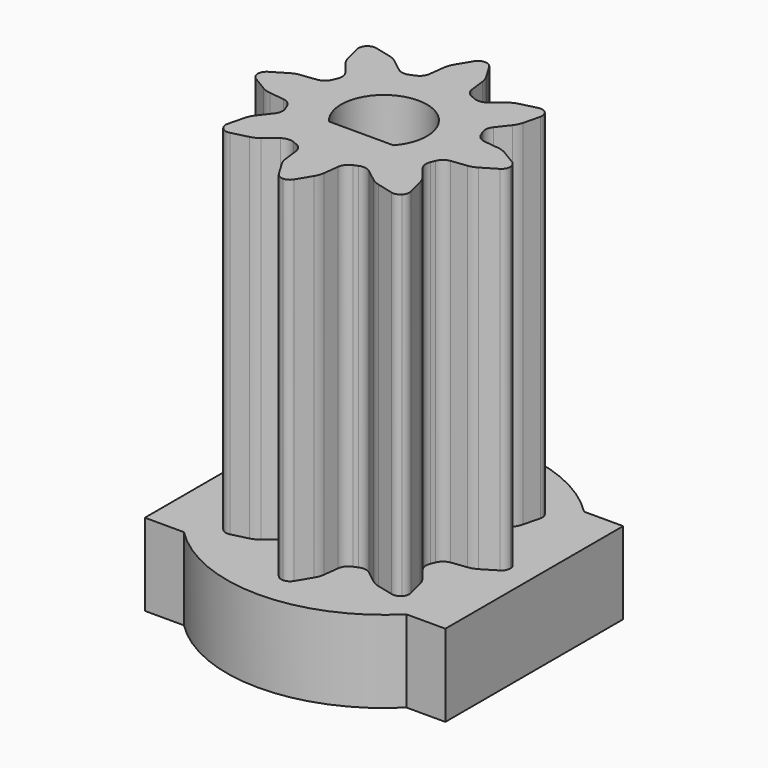
from build123d import *

# Parameters (mm, degrees)
F0_R     = 5
F0_R_2   = 3.15
F0_R_3   = 2.55
F1_DEPTH = 3.25
F2_R     = 2.55
F3_DEPTH = 14


# Not quite as in the source:
# - a feature names something its author has since deleted; it is built from what else it names


with BuildPart() as f1:
    # F0 (on Top) → F1 (new body)
    with BuildSketch(Plane.XY):
        with BuildLine():
            Line((-5.95, -4.4), (-4.4034787385, -4.4))
            ThreePointArc((-4.4034787385, -4.4), (0, -6.225), (4.4034787385, -4.4))
            Line((4.4034787385, -4.4), (5.95, -4.4))
            Line((5.95, -4.4), (5.95, 4.4))
            Line((5.95, 4.4), (4.4034787385, 4.4))
            ThreePointArc((4.4034787385, 4.4), (0, 6.225), (-4.4034787385, 4.4))
            Line((-4.4034787385, 4.4), (-5.95, 4.4))
            Line((-5.95, 4.4), (-5.95, -4.4))
        make_face()
        Circle(F0_R, mode=Mode.SUBTRACT)
        Circle(F0_R)
        Circle(F0_R_2, mode=Mode.SUBTRACT)
        Circle(F0_R_2)
        Circle(F0_R_3, mode=Mode.SUBTRACT)
        Circle(F0_R_3)
        with BuildLine():
            ThreePointArc((-1.275, -1.1244443072), (-0.601040764, 1.5902043894), (1.7, 0))
            ThreePointArc((1.7, 0), (1.5902043894, -0.601040764), (1.275, -1.1244443072))
            ThreePointArc((1.275, -1.1244443072), (0, -1.7), (-1.275, -1.1244443072))
        make_face(mode=Mode.SUBTRACT)
        with BuildLine():
            Line((1.275, -1.1244443072), (-1.275, -1.1244443072))
            ThreePointArc((-1.275, -1.1244443072), (0, -1.7), (1.275, -1.1244443072))
        make_face()
    extrude(amount=F1_DEPTH)

    # F2 (on face) → F3 (join)
    with BuildSketch(Plane.XY.offset(3.25)):
        with BuildLine():
            ThreePointArc((-4.8302633262, 0.3000085552), (-4.9546244936, 0.172348246), (-5, 0))
            ThreePointArc((-5, 0), (-4.9546244936, -0.172348246), (-4.8302633262, -0.3000085552))
            Line((-4.8302633262, -0.3000085552), (-4.2601369618, -0.6425750355))
            ThreePointArc((-4.2601369618, -0.6425750355), (-4.0929165173, -0.7205512094), (-3.9131380826, -0.7620563314))
            Line((-3.9131380826, -0.7620563314), (-3.3117988826, -0.835891501))
            ThreePointArc((-3.3117988826, -0.835891501), (-3.0868883315, -0.9291389359), (-2.9422567869, -1.125))
            ThreePointArc((-2.9422567869, -1.125), (-3.15, 0), (-2.9422567869, 1.125))
            ThreePointArc((-2.9422567869, 1.125), (-3.0868883315, 0.9291389359), (-3.3117988826, 0.835891501))
            Line((-3.3117988826, 0.835891501), (-3.9131380826, 0.7620563314))
            ThreePointArc((-3.9131380826, 0.7620563314), (-4.0929165173, 0.7205512094), (-4.2601369618, 0.6425750355))
            Line((-4.2601369618, 0.6425750355), (-4.8302633262, 0.3000085552))
        make_face()
        with BuildLine():
            ThreePointArc((-3.2033738691, 3.6276500367), (-3.3815799641, 3.6253171911), (-3.5355339059, 3.5355339059))
            ThreePointArc((-3.5355339059, 3.5355339059), (-3.6253171911, 3.3815799641), (-3.6276500367, 3.2033738691))
            Line((-3.6276500367, 3.2033738691), (-3.4667408995, 2.5580025694))
            ThreePointArc((-3.4667408995, 2.5580025694), (-3.4036356706, 2.3846223779), (-3.3058616735, 2.2281512744))
            Line((-3.3058616735, 2.2281512744), (-2.9328599965, 1.7507308991))
            ThreePointArc((-2.9328599965, 1.7507308991), (-2.8397601142, 1.5257592297), (-2.8759848548, 1.2849945972))
            ThreePointArc((-2.8759848548, 1.2849945972), (-2.2273863607, 2.2273863607), (-1.2849945972, 2.8759848548))
            ThreePointArc((-1.2849945972, 2.8759848548), (-1.5257592297, 2.8397601142), (-1.7507308991, 2.9328599965))
            Line((-1.7507308991, 2.9328599965), (-2.2281512744, 3.3058616735))
            ThreePointArc((-2.2281512744, 3.3058616735), (-2.3846223779, 3.4036356706), (-2.5580025694, 3.4667408995))
            Line((-2.5580025694, 3.4667408995), (-3.2033738691, 3.6276500367))
        make_face()
        with BuildLine():
            ThreePointArc((0.3000085552, 4.8302633262), (0.172348246, 4.9546244936), (0, 5))
            ThreePointArc((0, 5), (-0.172348246, 4.9546244936), (-0.3000085552, 4.8302633262))
            Line((-0.3000085552, 4.8302633262), (-0.6425750355, 4.2601369618))
            ThreePointArc((-0.6425750355, 4.2601369618), (-0.7205512094, 4.0929165173), (-0.7620563314, 3.9131380826))
            Line((-0.7620563314, 3.9131380826), (-0.835891501, 3.3117988826))
            ThreePointArc((-0.835891501, 3.3117988826), (-0.9291389359, 3.0868883315), (-1.125, 2.9422567869))
            ThreePointArc((-1.125, 2.9422567869), (0, 3.15), (1.125, 2.9422567869))
            ThreePointArc((1.125, 2.9422567869), (0.9291389359, 3.0868883315), (0.835891501, 3.3117988826))
            Line((0.835891501, 3.3117988826), (0.7620563314, 3.9131380826))
            ThreePointArc((0.7620563314, 3.9131380826), (0.7205512094, 4.0929165173), (0.6425750355, 4.2601369618))
            Line((0.6425750355, 4.2601369618), (0.3000085552, 4.8302633262))
        make_face()
        with BuildLine():
            ThreePointArc((3.2033738691, -3.6276500367), (3.3815799667, -3.6253171904), (3.5355339096, -3.5355339023))
            ThreePointArc((3.5355339096, -3.5355339023), (3.6253171918, -3.3815799616), (3.6276500367, -3.2033738691))
            Line((3.6276500367, -3.2033738691), (3.4667408995, -2.5580025694))
            ThreePointArc((3.4667408995, -2.5580025694), (3.4036356706, -2.3846223779), (3.3058616735, -2.2281512744))
            Line((3.3058616735, -2.2281512744), (2.9328599965, -1.7507308991))
            ThreePointArc((2.9328599965, -1.7507308991), (2.8397601142, -1.5257592297), (2.8759848548, -1.2849945972))
            ThreePointArc((2.8759848548, -1.2849945972), (2.2273863607, -2.2273863607), (1.2849945972, -2.8759848548))
            ThreePointArc((1.2849945972, -2.8759848548), (1.5257592297, -2.8397601142), (1.7507308991, -2.9328599965))
            Line((1.7507308991, -2.9328599965), (2.2281512744, -3.3058616735))
            ThreePointArc((2.2281512744, -3.3058616735), (2.3846223779, -3.4036356706), (2.5580025694, -3.4667408995))
            Line((2.5580025694, -3.4667408995), (3.2033738691, -3.6276500367))
        make_face()
        with BuildLine():
            ThreePointArc((-0.3000085552, -4.8302633262), (-0.172348246, -4.9546244936), (0, -5))
            ThreePointArc((0, -5), (0.172348246, -4.9546244936), (0.3000085552, -4.8302633262))
            Line((0.3000085552, -4.8302633262), (0.6425750355, -4.2601369618))
            ThreePointArc((0.6425750355, -4.2601369618), (0.7205512094, -4.0929165173), (0.7620563314, -3.9131380826))
            Line((0.7620563314, -3.9131380826), (0.835891501, -3.3117988826))
            ThreePointArc((0.835891501, -3.3117988826), (0.9291389359, -3.0868883315), (1.125, -2.9422567869))
            ThreePointArc((1.125, -2.9422567869), (0, -3.15), (-1.125, -2.9422567869))
            ThreePointArc((-1.125, -2.9422567869), (-0.9291389359, -3.0868883315), (-0.835891501, -3.3117988826))
            Line((-0.835891501, -3.3117988826), (-0.7620563314, -3.9131380826))
            ThreePointArc((-0.7620563314, -3.9131380826), (-0.7205512094, -4.0929165173), (-0.6425750355, -4.2601369618))
            Line((-0.6425750355, -4.2601369618), (-0.3000085552, -4.8302633262))
        make_face()
        with BuildLine():
            ThreePointArc((-3.6276500367, -3.2033738691), (-3.6253171911, -3.3815799641), (-3.5355339059, -3.5355339059))
            ThreePointArc((-3.5355339059, -3.5355339059), (-3.3815799641, -3.6253171911), (-3.2033738691, -3.6276500367))
            Line((-3.2033738691, -3.6276500367), (-2.5580025694, -3.4667408995))
            ThreePointArc((-2.5580025694, -3.4667408995), (-2.3846223779, -3.4036356706), (-2.2281512744, -3.3058616735))
            Line((-2.2281512744, -3.3058616735), (-1.7507308991, -2.9328599965))
            ThreePointArc((-1.7507308991, -2.9328599965), (-1.5257592297, -2.8397601142), (-1.2849945972, -2.8759848548))
            ThreePointArc((-1.2849945972, -2.8759848548), (-2.2273863607, -2.2273863607), (-2.8759848548, -1.2849945972))
            ThreePointArc((-2.8759848548, -1.2849945972), (-2.8397601142, -1.5257592297), (-2.9328599965, -1.7507308991))
            Line((-2.9328599965, -1.7507308991), (-3.3058616735, -2.2281512744))
            ThreePointArc((-3.3058616735, -2.2281512744), (-3.4036356706, -2.3846223779), (-3.4667408995, -2.5580025694))
            Line((-3.4667408995, -2.5580025694), (-3.6276500367, -3.2033738691))
        make_face()
        with BuildLine():
            ThreePointArc((2.8759848548, -1.2849945972), (2.9102205274, -1.205452812), (2.9422567869, -1.125))
            ThreePointArc((2.9422567869, -1.125), (3.0976288414, -0.5720101054), (3.15, 0))
            ThreePointArc((3.15, 0), (3.0976288414, 0.5720101054), (2.9422567869, 1.125))
            ThreePointArc((2.9422567869, 1.125), (2.9102205274, 1.205452812), (2.8759848548, 1.2849945972))
            ThreePointArc((2.8759848548, 1.2849945972), (2.2273863607, 2.2273863607), (1.2849945972, 2.8759848548))
            ThreePointArc((1.2849945972, 2.8759848548), (1.205452812, 2.9102205274), (1.125, 2.9422567869))
            ThreePointArc((1.125, 2.9422567869), (0, 3.15), (-1.125, 2.9422567869))
            ThreePointArc((-1.125, 2.9422567869), (-1.205452812, 2.9102205274), (-1.2849945972, 2.8759848548))
            ThreePointArc((-1.2849945972, 2.8759848548), (-2.2273863607, 2.2273863607), (-2.8759848548, 1.2849945972))
            ThreePointArc((-2.8759848548, 1.2849945972), (-2.9102205274, 1.205452812), (-2.9422567869, 1.125))
            ThreePointArc((-2.9422567869, 1.125), (-3.15, 0), (-2.9422567869, -1.125))
            ThreePointArc((-2.9422567869, -1.125), (-2.9102205274, -1.205452812), (-2.8759848548, -1.2849945972))
            ThreePointArc((-2.8759848548, -1.2849945972), (-2.2273863607, -2.2273863607), (-1.2849945972, -2.8759848548))
            ThreePointArc((-1.2849945972, -2.8759848548), (-1.205452812, -2.9102205274), (-1.125, -2.9422567869))
            ThreePointArc((-1.125, -2.9422567869), (0, -3.15), (1.125, -2.9422567869))
            ThreePointArc((1.125, -2.9422567869), (1.205452812, -2.9102205274), (1.2849945972, -2.8759848548))
            ThreePointArc((1.2849945972, -2.8759848548), (2.2273863607, -2.2273863607), (2.8759848548, -1.2849945972))
        make_face()
        Circle(F2_R, mode=Mode.SUBTRACT)
        Circle(F2_R)
        with BuildLine():
            Line((1.275, -1.1244443072), (-1.275, -1.1244443072))
            ThreePointArc((-1.275, -1.1244443072), (0, 1.7), (1.275, -1.1244443072))
        make_face(mode=Mode.SUBTRACT)
        with BuildLine():
            ThreePointArc((3.6276500367, 3.2033738691), (3.6253171915, 3.3815799629), (3.5355339078, 3.5355339041))
            ThreePointArc((3.5355339078, 3.5355339041), (3.3815799654, 3.6253171908), (3.2033738691, 3.6276500367))
            Line((3.2033738691, 3.6276500367), (2.5580025694, 3.4667408995))
            ThreePointArc((2.5580025694, 3.4667408995), (2.3846223779, 3.4036356706), (2.2281512744, 3.3058616735))
            Line((2.2281512744, 3.3058616735), (1.7507308991, 2.9328599965))
            ThreePointArc((1.7507308991, 2.9328599965), (1.5257592297, 2.8397601142), (1.2849945972, 2.8759848548))
            ThreePointArc((1.2849945972, 2.8759848548), (2.2273863607, 2.2273863607), (2.8759848548, 1.2849945972))
            ThreePointArc((2.8759848548, 1.2849945972), (2.8397601142, 1.5257592297), (2.9328599965, 1.7507308991))
            Line((2.9328599965, 1.7507308991), (3.3058616735, 2.2281512744))
            ThreePointArc((3.3058616735, 2.2281512744), (3.4036356706, 2.3846223779), (3.4667408995, 2.5580025694))
            Line((3.4667408995, 2.5580025694), (3.6276500367, 3.2033738691))
        make_face()
        with BuildLine():
            ThreePointArc((4.8302633262, -0.3000085552), (4.9546244936, -0.172348246), (5, 0))
            ThreePointArc((5, 0), (4.9546244936, 0.172348246), (4.8302633262, 0.3000085552))
            Line((4.8302633262, 0.3000085552), (4.2601369618, 0.6425750355))
            ThreePointArc((4.2601369618, 0.6425750355), (4.0929165173, 0.7205512094), (3.9131380826, 0.7620563314))
            Line((3.9131380826, 0.7620563314), (3.3117988826, 0.835891501))
            ThreePointArc((3.3117988826, 0.835891501), (3.0868883315, 0.9291389359), (2.9422567869, 1.125))
            ThreePointArc((2.9422567869, 1.125), (3.0976288414, 0.5720101054), (3.15, 0))
            ThreePointArc((3.15, 0), (3.0976288414, -0.5720101054), (2.9422567869, -1.125))
            ThreePointArc((2.9422567869, -1.125), (3.0868883315, -0.9291389359), (3.3117988826, -0.835891501))
            Line((3.3117988826, -0.835891501), (3.9131380826, -0.7620563314))
            ThreePointArc((3.9131380826, -0.7620563314), (4.0929165173, -0.7205512094), (4.2601369618, -0.6425750355))
            Line((4.2601369618, -0.6425750355), (4.8302633262, -0.3000085552))
        make_face()
    extrude(amount=F3_DEPTH)


solid = f1.part
